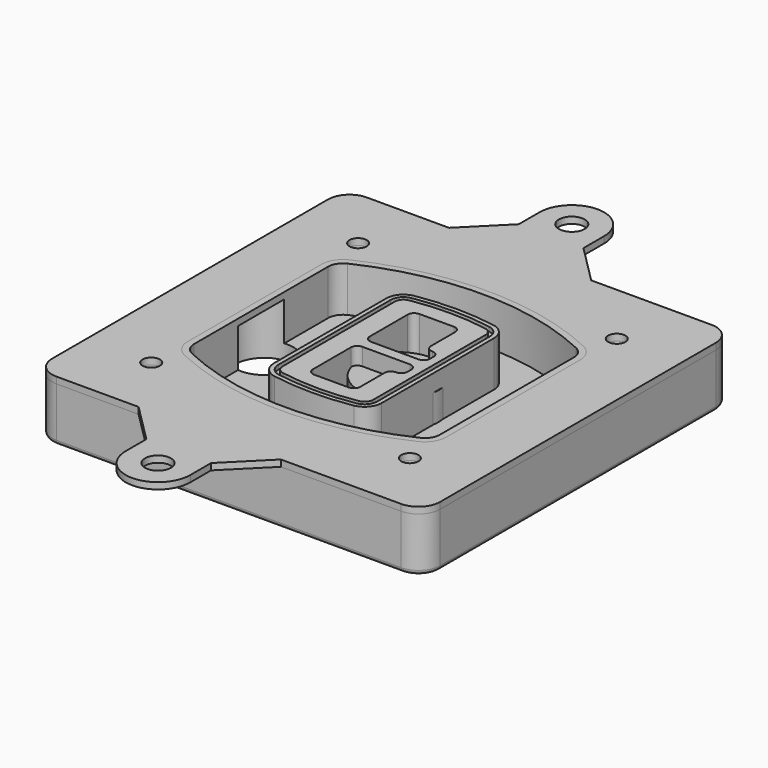
from build123d import *

# Parameters (mm, degrees)
F0_R      = 4
F1_DEPTH  = 25
F2_DEPTH  = 3
F3_DEPTH  = 18
F5_DEPTH  = 21
F6_DEPTH  = 2
F8_DEPTH  = 20
F9_DEPTH  = 16
F10_DEPTH = 25
F7_R      = 6
F7_R_2    = 4
F11_DEPTH = 6
F13_DEPTH = 9
F15_R     = 2
F16_R     = 4
F16_R_2   = 6
F17_DEPTH = 3


# Not quite as in the source:
# - a feature of the source that left no trace in its solid (it failed there, or was rolled back) is left out
# - a feature names something its author has since deleted; it is built from what else it names


with BuildPart() as f1:
    # F0 (on Top) → F1 (new body)
    with BuildSketch(Plane.XY):
        with BuildLine():
            ThreePointArc((-90, -80), (-87.0710678119, -87.0710678119), (-80, -90))
            Line((-80, -90), (80, -90))
            ThreePointArc((80, -90), (87.0710678119, -87.0710678119), (90, -80))
            Line((90, -80), (90, 80))
            ThreePointArc((90, 80), (87.0710678119, 87.0710678119), (80, 90))
            Line((80, 90), (-80, 90))
            ThreePointArc((-80, 90), (-87.0710678119, 87.0710678119), (-90, 80))
            Line((-90, 80), (-90, -80))
        make_face()
        with Locations((-60, -60)):
            Circle(F0_R, mode=Mode.SUBTRACT)
        with Locations((60, -60)):
            Circle(F0_R, mode=Mode.SUBTRACT)
        with BuildLine():
            ThreePointArc((-64, 38.8308515907), (-61.8195654598, 46.3340424013), (-55.9574468085, 51.5000594398))
            ThreePointArc((-55.9574468085, 51.5000594398), (0, 64), (55.9574468085, 51.5000594398))
            ThreePointArc((55.9574468085, 51.5000594398), (61.8195654598, 46.3340424013), (64, 38.8308515907))
            Line((64, 38.8308515907), (64, -38.8308515907))
            ThreePointArc((64, -38.8308515907), (61.8195654598, -46.3340424013), (55.9574468085, -51.5000594398))
            ThreePointArc((55.9574468085, -51.5000594398), (0, -64), (-55.9574468085, -51.5000594398))
            ThreePointArc((-55.9574468085, -51.5000594398), (-61.8195654598, -46.3340424013), (-64, -38.8308515907))
            Line((-64, -38.8308515907), (-64, 38.8308515907))
        make_face(mode=Mode.SUBTRACT)
        with Locations((-60, 60)):
            Circle(F0_R, mode=Mode.SUBTRACT)
        with Locations((60, 60)):
            Circle(F0_R, mode=Mode.SUBTRACT)
        with BuildLine():
            ThreePointArc((55.9574468085, 51.5000594398), (0, 64), (-55.9574468085, 51.5000594398))
            ThreePointArc((-55.9574468085, 51.5000594398), (-61.8195654598, 46.3340424013), (-64, 38.8308515907))
            Line((-64, 38.8308515907), (-64, -38.8308515907))
            ThreePointArc((-64, -38.8308515907), (-61.8195654598, -46.3340424013), (-55.9574468085, -51.5000594398))
            ThreePointArc((-55.9574468085, -51.5000594398), (0, -64), (55.9574468085, -51.5000594398))
            ThreePointArc((55.9574468085, -51.5000594398), (61.8195654598, -46.3340424013), (64, -38.8308515907))
            Line((64, -38.8308515907), (64, 38.8308515907))
            ThreePointArc((64, 38.8308515907), (61.8195654598, 46.3340424013), (55.9574468085, 51.5000594398))
        make_face()
        with BuildLine():
            Line((-60, -38.8308515907), (-60, 38.8308515907))
            ThreePointArc((-60, 38.8308515907), (-58.442546757, 44.1902735983), (-54.2553191489, 47.8802857686))
            ThreePointArc((-54.2553191489, 47.8802857686), (0, 60), (54.2553191489, 47.8802857686))
            ThreePointArc((54.2553191489, 47.8802857686), (58.442546757, 44.1902735983), (60, 38.8308515907))
            Line((60, 38.8308515907), (60, -38.8308515907))
            ThreePointArc((60, -38.8308515907), (58.442546757, -44.1902735983), (54.2553191489, -47.8802857686))
            ThreePointArc((54.2553191489, -47.8802857686), (0, -60), (-54.2553191489, -47.8802857686))
            ThreePointArc((-54.2553191489, -47.8802857686), (-58.442546757, -44.1902735983), (-60, -38.8308515907))
        make_face(mode=Mode.SUBTRACT)
        with BuildLine():
            ThreePointArc((-54.2553191489, 47.8802857686), (-58.442546757, 44.1902735983), (-60, 38.8308515907))
            Line((-60, 38.8308515907), (-60, -38.8308515907))
            ThreePointArc((-60, -38.8308515907), (-58.442546757, -44.1902735983), (-54.2553191489, -47.8802857686))
            ThreePointArc((-54.2553191489, -47.8802857686), (0, -60), (54.2553191489, -47.8802857686))
            ThreePointArc((54.2553191489, -47.8802857686), (58.442546757, -44.1902735983), (60, -38.8308515907))
            Line((60, -38.8308515907), (60, 38.8308515907))
            ThreePointArc((60, 38.8308515907), (58.442546757, 44.1902735983), (54.2553191489, 47.8802857686))
            ThreePointArc((54.2553191489, 47.8802857686), (0, 60), (-54.2553191489, 47.8802857686))
        make_face()
        with BuildLine():
            ThreePointArc((52.9787234043, 45.1654555152), (55.9097827299, 42.582446996), (57, 38.8308515907))
            Line((57, 38.8308515907), (57, -38.8308515907))
            ThreePointArc((57, -38.8308515907), (55.9097827299, -42.582446996), (52.9787234043, -45.1654555152))
            ThreePointArc((52.9787234043, -45.1654555152), (0, -57), (-52.9787234043, -45.1654555152))
            ThreePointArc((-52.9787234043, -45.1654555152), (-55.9097827299, -42.582446996), (-57, -38.8308515907))
            Line((-57, -38.8308515907), (-57, 38.8308515907))
            ThreePointArc((-57, 38.8308515907), (-55.9097827299, 42.582446996), (-52.9787234043, 45.1654555152))
            ThreePointArc((-52.9787234043, 45.1654555152), (0, 57), (52.9787234043, 45.1654555152))
        make_face(mode=Mode.SUBTRACT)
        with BuildLine():
            Line((57, -38.8308515907), (57, 38.8308515907))
            ThreePointArc((57, 38.8308515907), (55.9097827299, 42.582446996), (52.9787234043, 45.1654555152))
            ThreePointArc((52.9787234043, 45.1654555152), (0, 57), (-52.9787234043, 45.1654555152))
            ThreePointArc((-52.9787234043, 45.1654555152), (-55.9097827299, 42.582446996), (-57, 38.8308515907))
            Line((-57, 38.8308515907), (-57, -38.8308515907))
            ThreePointArc((-57, -38.8308515907), (-55.9097827299, -42.582446996), (-52.9787234043, -45.1654555152))
            ThreePointArc((-52.9787234043, -45.1654555152), (0, -57), (52.9787234043, -45.1654555152))
            ThreePointArc((52.9787234043, -45.1654555152), (55.9097827299, -42.582446996), (57, -38.8308515907))
        make_face()
    extrude(amount=-F1_DEPTH)

    # F0 (on Top) → F2 (join)
    with BuildSketch(Plane.XY):
        with BuildLine():
            ThreePointArc((-54.2553191489, 47.8802857686), (-58.442546757, 44.1902735983), (-60, 38.8308515907))
            Line((-60, 38.8308515907), (-60, -38.8308515907))
            ThreePointArc((-60, -38.8308515907), (-58.442546757, -44.1902735983), (-54.2553191489, -47.8802857686))
            ThreePointArc((-54.2553191489, -47.8802857686), (0, -60), (54.2553191489, -47.8802857686))
            ThreePointArc((54.2553191489, -47.8802857686), (58.442546757, -44.1902735983), (60, -38.8308515907))
            Line((60, -38.8308515907), (60, 38.8308515907))
            ThreePointArc((60, 38.8308515907), (58.442546757, 44.1902735983), (54.2553191489, 47.8802857686))
            ThreePointArc((54.2553191489, 47.8802857686), (0, 60), (-54.2553191489, 47.8802857686))
        make_face()
        with BuildLine():
            ThreePointArc((52.9787234043, 45.1654555152), (55.9097827299, 42.582446996), (57, 38.8308515907))
            Line((57, 38.8308515907), (57, -38.8308515907))
            ThreePointArc((57, -38.8308515907), (55.9097827299, -42.582446996), (52.9787234043, -45.1654555152))
            ThreePointArc((52.9787234043, -45.1654555152), (0, -57), (-52.9787234043, -45.1654555152))
            ThreePointArc((-52.9787234043, -45.1654555152), (-55.9097827299, -42.582446996), (-57, -38.8308515907))
            Line((-57, -38.8308515907), (-57, 38.8308515907))
            ThreePointArc((-57, 38.8308515907), (-55.9097827299, 42.582446996), (-52.9787234043, 45.1654555152))
            ThreePointArc((-52.9787234043, 45.1654555152), (0, 57), (52.9787234043, 45.1654555152))
        make_face(mode=Mode.SUBTRACT)
    extrude(amount=F2_DEPTH)

    # F0 (on Top) → F3 (cut)
    with BuildSketch(Plane.XY):
        with BuildLine():
            Line((57, -38.8308515907), (57, 38.8308515907))
            ThreePointArc((57, 38.8308515907), (55.9097827299, 42.582446996), (52.9787234043, 45.1654555152))
            ThreePointArc((52.9787234043, 45.1654555152), (0, 57), (-52.9787234043, 45.1654555152))
            ThreePointArc((-52.9787234043, 45.1654555152), (-55.9097827299, 42.582446996), (-57, 38.8308515907))
            Line((-57, 38.8308515907), (-57, -38.8308515907))
            ThreePointArc((-57, -38.8308515907), (-55.9097827299, -42.582446996), (-52.9787234043, -45.1654555152))
            ThreePointArc((-52.9787234043, -45.1654555152), (0, -57), (52.9787234043, -45.1654555152))
            ThreePointArc((52.9787234043, -45.1654555152), (55.9097827299, -42.582446996), (57, -38.8308515907))
        make_face()
    extrude(amount=-F3_DEPTH, mode=Mode.SUBTRACT)

    # F4 (on face) → F5 (join, through all)
    with BuildSketch(Plane.XY.offset(3)):
        with BuildLine():
            ThreePointArc((-25, -32.5662280692), (-23.1122504785, -37.7276614059), (-18.3399014778, -40.4532214146))
            ThreePointArc((-18.3399014778, -40.4532214146), (0, -42), (18.3399014778, -40.4532214146))
            ThreePointArc((18.3399014778, -40.4532214146), (23.1122504785, -37.7276614059), (25, -32.5662280692))
            Line((25, -32.5662280692), (25, 32.5662280692))
            ThreePointArc((25, 32.5662280692), (23.1122504785, 37.7276614059), (18.3399014778, 40.4532214146))
            ThreePointArc((18.3399014778, 40.4532214146), (0, 42), (-18.3399014778, 40.4532214146))
            ThreePointArc((-18.3399014778, 40.4532214146), (-23.1122504785, 37.7276614059), (-25, 32.5662280692))
            Line((-25, 32.5662280692), (-25, -32.5662280692))
        make_face()
        with BuildLine():
            ThreePointArc((18.0049261084, 38.4814730782), (21.5841878588, 36.4373030717), (23, 32.5662280692))
            Line((23, 32.5662280692), (23, -32.5662280692))
            ThreePointArc((23, -32.5662280692), (21.5841878588, -36.4373030717), (18.0049261084, -38.4814730782))
            ThreePointArc((18.0049261084, -38.4814730782), (0, -40), (-18.0049261084, -38.4814730782))
            ThreePointArc((-18.0049261084, -38.4814730782), (-21.5841878588, -36.4373030717), (-23, -32.5662280692))
            Line((-23, -32.5662280692), (-23, 32.5662280692))
            ThreePointArc((-23, 32.5662280692), (-21.5841878588, 36.4373030717), (-18.0049261084, 38.4814730782))
            ThreePointArc((-18.0049261084, 38.4814730782), (0, 40), (18.0049261084, 38.4814730782))
        make_face(mode=Mode.SUBTRACT)
        with BuildLine():
            Line((23, -32.5662280692), (23, 32.5662280692))
            ThreePointArc((23, 32.5662280692), (21.5841878588, 36.4373030717), (18.0049261084, 38.4814730782))
            ThreePointArc((18.0049261084, 38.4814730782), (0, 40), (-18.0049261084, 38.4814730782))
            ThreePointArc((-18.0049261084, 38.4814730782), (-21.5841878588, 36.4373030717), (-23, 32.5662280692))
            Line((-23, 32.5662280692), (-23, -32.5662280692))
            ThreePointArc((-23, -32.5662280692), (-21.5841878588, -36.4373030717), (-18.0049261084, -38.4814730782))
            ThreePointArc((-18.0049261084, -38.4814730782), (0, -40), (18.0049261084, -38.4814730782))
            ThreePointArc((18.0049261084, -38.4814730782), (21.5841878588, -36.4373030717), (23, -32.5662280692))
        make_face()
        with BuildLine():
            ThreePointArc((17.6699507389, 36.5097247419), (20.0561252392, 35.1469447375), (21, 32.5662280692))
            Line((21, 32.5662280692), (21, -32.5662280692))
            ThreePointArc((21, -32.5662280692), (20.0561252392, -35.1469447375), (17.6699507389, -36.5097247419))
            ThreePointArc((17.6699507389, -36.5097247419), (0, -38), (-17.6699507389, -36.5097247419))
            ThreePointArc((-17.6699507389, -36.5097247419), (-20.0561252392, -35.1469447375), (-21, -32.5662280692))
            Line((-21, -32.5662280692), (-21, 32.5662280692))
            ThreePointArc((-21, 32.5662280692), (-20.0561252392, 35.1469447375), (-17.6699507389, 36.5097247419))
            ThreePointArc((-17.6699507389, 36.5097247419), (0, 38), (17.6699507389, 36.5097247419))
        make_face(mode=Mode.SUBTRACT)
        with BuildLine():
            Line((21, -32.5662280692), (21, 32.5662280692))
            ThreePointArc((21, 32.5662280692), (20.0561252392, 35.1469447375), (17.6699507389, 36.5097247419))
            ThreePointArc((17.6699507389, 36.5097247419), (0, 38), (-17.6699507389, 36.5097247419))
            ThreePointArc((-17.6699507389, 36.5097247419), (-20.0561252392, 35.1469447375), (-21, 32.5662280692))
            Line((-21, 32.5662280692), (-21, -32.5662280692))
            ThreePointArc((-21, -32.5662280692), (-20.0561252392, -35.1469447375), (-17.6699507389, -36.5097247419))
            ThreePointArc((-17.6699507389, -36.5097247419), (0, -38), (17.6699507389, -36.5097247419))
            ThreePointArc((17.6699507389, -36.5097247419), (20.0561252392, -35.1469447375), (21, -32.5662280692))
        make_face()
        with BuildLine():
            Line((-8, -2.5), (14, -2.5))
            ThreePointArc((14, -2.5), (16.1213203436, -3.3786796564), (17, -5.5))
            Line((17, -5.5), (17, -7.5))
            ThreePointArc((17, -7.5), (16.1213203436, -9.6213203436), (14, -10.5))
            ThreePointArc((14, -10.5), (11.8786796564, -11.3786796564), (11, -13.5))
            Line((11, -13.5), (11, -27.5))
            ThreePointArc((11, -27.5), (10.1213203436, -29.6213203436), (8, -30.5))
            Line((8, -30.5), (-8, -30.5))
            ThreePointArc((-8, -30.5), (-10.1213203436, -29.6213203436), (-11, -27.5))
            Line((-11, -27.5), (-11, -5.5))
            ThreePointArc((-11, -5.5), (-10.1213203436, -3.3786796564), (-8, -2.5))
        make_face(mode=Mode.SUBTRACT)
        with BuildLine():
            ThreePointArc((-8, 2.5), (-10.1213203436, 3.3786796564), (-11, 5.5))
            Line((-11, 5.5), (-11, 27.5))
            ThreePointArc((-11, 27.5), (-10.1213203436, 29.6213203436), (-8, 30.5))
            Line((-8, 30.5), (8, 30.5))
            ThreePointArc((8, 30.5), (10.1213203436, 29.6213203436), (11, 27.5))
            Line((11, 27.5), (11, 13.5))
            ThreePointArc((11, 13.5), (11.8786796564, 11.3786796564), (14, 10.5))
            ThreePointArc((14, 10.5), (16.1213203436, 9.6213203436), (17, 7.5))
            Line((17, 7.5), (17, 5.5))
            ThreePointArc((17, 5.5), (16.1213203436, 3.3786796564), (14, 2.5))
            Line((14, 2.5), (-8, 2.5))
        make_face(mode=Mode.SUBTRACT)
    extrude(amount=-F5_DEPTH)

    # F4 (on face) → F6 (cut)
    with BuildSketch(Plane.XY.offset(3)):
        with BuildLine():
            Line((23, -32.5662280692), (23, 32.5662280692))
            ThreePointArc((23, 32.5662280692), (21.5841878588, 36.4373030717), (18.0049261084, 38.4814730782))
            ThreePointArc((18.0049261084, 38.4814730782), (0, 40), (-18.0049261084, 38.4814730782))
            ThreePointArc((-18.0049261084, 38.4814730782), (-21.5841878588, 36.4373030717), (-23, 32.5662280692))
            Line((-23, 32.5662280692), (-23, -32.5662280692))
            ThreePointArc((-23, -32.5662280692), (-21.5841878588, -36.4373030717), (-18.0049261084, -38.4814730782))
            ThreePointArc((-18.0049261084, -38.4814730782), (0, -40), (18.0049261084, -38.4814730782))
            ThreePointArc((18.0049261084, -38.4814730782), (21.5841878588, -36.4373030717), (23, -32.5662280692))
        make_face()
        with BuildLine():
            ThreePointArc((17.6699507389, 36.5097247419), (20.0561252392, 35.1469447375), (21, 32.5662280692))
            Line((21, 32.5662280692), (21, -32.5662280692))
            ThreePointArc((21, -32.5662280692), (20.0561252392, -35.1469447375), (17.6699507389, -36.5097247419))
            ThreePointArc((17.6699507389, -36.5097247419), (0, -38), (-17.6699507389, -36.5097247419))
            ThreePointArc((-17.6699507389, -36.5097247419), (-20.0561252392, -35.1469447375), (-21, -32.5662280692))
            Line((-21, -32.5662280692), (-21, 32.5662280692))
            ThreePointArc((-21, 32.5662280692), (-20.0561252392, 35.1469447375), (-17.6699507389, 36.5097247419))
            ThreePointArc((-17.6699507389, 36.5097247419), (0, 38), (17.6699507389, 36.5097247419))
        make_face(mode=Mode.SUBTRACT)
    extrude(amount=-F6_DEPTH, mode=Mode.SUBTRACT)

    # F7 (on face) → F8 (join)
    with BuildSketch(Plane(origin=(0, 0, -25), x_dir=(1, 0, 0), z_dir=(0, 0, -1))):
        with BuildLine():
            ThreePointArc((-6.71157564, 0), (6.7567035675, 13.4682792075), (20.224982775, 0))
            Line((20.224982775, 0), (25.224982775, 0))
            ThreePointArc((25.224982775, 0), (6.7567035675, 18.4682792075), (-11.71157564, 0))
            Line((-11.71157564, 0), (-6.71157564, 0))
        make_face()
        with BuildLine():
            Line((-6.71157564, 0), (20.224982775, 0))
            ThreePointArc((20.224982775, 0), (6.7567035675, 13.4682792075), (-6.71157564, 0))
        make_face()
        with BuildLine():
            ThreePointArc((-6.71157564, 0), (6.7567035675, -13.4682792075), (20.224982775, 0))
            Line((20.224982775, 0), (-6.71157564, 0))
        make_face()
        with BuildLine():
            Line((25.224982775, 0), (20.224982775, 0))
            ThreePointArc((20.224982775, 0), (6.7567035675, -13.4682792075), (-6.71157564, 0))
            Line((-6.71157564, 0), (-11.71157564, 0))
            ThreePointArc((-11.71157564, 0), (6.7567035675, -18.4682792075), (25.224982775, 0))
        make_face()
    extrude(amount=-F8_DEPTH)

    # F7 (on face) → F9 (cut)
    with BuildSketch(Plane(origin=(0, 0, -25), x_dir=(1, 0, 0), z_dir=(0, 0, -1))):
        with BuildLine():
            Line((-6.71157564, 0), (20.224982775, 0))
            ThreePointArc((20.224982775, 0), (6.7567035675, 13.4682792075), (-6.71157564, 0))
        make_face()
        with BuildLine():
            ThreePointArc((-6.71157564, 0), (6.7567035675, -13.4682792075), (20.224982775, 0))
            Line((20.224982775, 0), (-6.71157564, 0))
        make_face()
    extrude(amount=-F9_DEPTH, mode=Mode.SUBTRACT)

    # F7 (on face) → F10 (cut)
    with BuildSketch(Plane(origin=(0, 0, -25), x_dir=(1, 0, 0), z_dir=(0, 0, -1))):
        with BuildLine():
            Line((-69.0318229325, 0), (-42.0952645175, 0))
            ThreePointArc((-42.0952645175, 0), (-55.563543725, 13.4682792075), (-69.0318229325, 0))
        make_face()
        with BuildLine():
            ThreePointArc((-69.0318229325, 0), (-55.563543725, -13.4682792075), (-42.0952645175, 0))
            Line((-42.0952645175, 0), (-69.0318229325, 0))
        make_face()
    extrude(amount=-F10_DEPTH, mode=Mode.SUBTRACT)

    # F7 (on face) → F11 (cut)
    with BuildSketch(Plane(origin=(0, 0, -25), x_dir=(1, 0, 0), z_dir=(0, 0, -1))):
        with Locations((60, -60)):
            Circle(F7_R)
        with Locations((60, -60)):
            Circle(F7_R_2, mode=Mode.SUBTRACT)
        with Locations((-60, -60)):
            Circle(F7_R)
        with Locations((-60, -60)):
            Circle(F7_R_2, mode=Mode.SUBTRACT)
        with Locations((-60, 60)):
            Circle(F7_R)
        with Locations((-60, 60)):
            Circle(F7_R_2, mode=Mode.SUBTRACT)
        with Locations((60, 60)):
            Circle(F7_R)
        with Locations((60, 60)):
            Circle(F7_R_2, mode=Mode.SUBTRACT)
    extrude(amount=-F11_DEPTH, mode=Mode.SUBTRACT)

    # F12 (on face) → F13 (cut, through all)
    with BuildSketch(Plane(origin=(0, 0, -9), x_dir=(1, 0, 0), z_dir=(0, 0, -1))):
        with BuildLine():
            ThreePointArc((20.224982775, 0), (20.1663399806, 1.2554664788), (19.9909222755, 2.5))
            Line((19.9909222755, 2.5), (14, 2.5))
            ThreePointArc((14, 2.5), (16.1213203436, 3.3786796564), (17, 5.5))
            Line((17, 5.5), (17, 7.5))
            ThreePointArc((17, 7.5), (16.1213203436, 9.6213203436), (14, 10.5))
            ThreePointArc((14, 10.5), (12.1627255951, 11.1284134507), (11.0951631559, 12.750384826))
            ThreePointArc((11.0951631559, 12.750384826), (11.0476113807, 12.7664660322), (11, 12.7823698976))
            Line((11, 12.7823698976), (11, -12.7823698976))
            ThreePointArc((11, -12.7823698976), (11.0476113807, -12.7664660322), (11.0951631559, -12.750384826))
            ThreePointArc((11.0951631559, -12.750384826), (12.1627255951, -11.1284134507), (14, -10.5))
            ThreePointArc((14, -10.5), (16.1213203436, -9.6213203436), (17, -7.5))
            Line((17, -7.5), (17, -5.5))
            ThreePointArc((17, -5.5), (16.1213203436, -3.3786796564), (14, -2.5))
            Line((14, -2.5), (19.9909222755, -2.5))
            ThreePointArc((19.9909222755, -2.5), (20.1663399806, -1.2554664788), (20.224982775, 0))
        make_face()
    extrude(amount=F13_DEPTH, mode=Mode.SUBTRACT)

    # F15
    f15_edges = [f1.edges().sort_by_distance(p)[0] for p in [
        (0, -90, -25),
        (-87.071068, -87.071068, -25),
        (-90, 0, -25),
        (-87.071068, 87.071068, -25),
        (87.071068, -87.071068, -25),
        (0, 90, -25),
        (90, 0, -25),
        (87.071068, 87.071068, -25),
    ]]
    fillet(f15_edges, radius=F15_R)


with BuildPart() as f17:
    # F16 (on Top) → F17 (new body, through all)
    with BuildSketch(Plane.XY):
        with BuildLine():
            Line((-90, 80), (-90, -80))
            ThreePointArc((-90, -80), (-87.0710678119, -87.0710678119), (-80, -90))
            Line((-80, -90), (-41.8600961566, -90))
            Line((-41.8600961566, -90), (24.1399038434, -90))
            Line((24.1399038434, -90), (80, -90))
            ThreePointArc((80, -90), (87.0710678119, -87.0710678119), (90, -80))
            Line((90, -80), (90, 80))
            ThreePointArc((90, 80), (87.0710678119, 87.0710678119), (80, 90))
            Line((80, 90), (24.1399038434, 90))
            Line((24.1399038434, 90), (-41.8600961566, 90))
            Line((-41.8600961566, 90), (-80, 90))
            ThreePointArc((-80, 90), (-87.0710678119, 87.0710678119), (-90, 80))
        make_face()
        with Locations((-60, -60)):
            Circle(F16_R, mode=Mode.SUBTRACT)
        with Locations((60, -60)):
            Circle(F16_R, mode=Mode.SUBTRACT)
        with Locations((-60, 60)):
            Circle(F16_R, mode=Mode.SUBTRACT)
        with BuildLine():
            ThreePointArc((-54.2553191489, 47.8802857686), (0, 60), (54.2553191489, 47.8802857686))
            ThreePointArc((54.2553191489, 47.8802857686), (58.442546757, 44.1902735983), (60, 38.8308515907))
            Line((60, 38.8308515907), (60, -38.8308515907))
            ThreePointArc((60, -38.8308515907), (58.442546757, -44.1902735983), (54.2553191489, -47.8802857686))
            ThreePointArc((54.2553191489, -47.8802857686), (0, -60), (-54.2553191489, -47.8802857686))
            ThreePointArc((-54.2553191489, -47.8802857686), (-58.442546757, -44.1902735983), (-60, -38.8308515907))
            Line((-60, -38.8308515907), (-60, 38.8308515907))
            ThreePointArc((-60, 38.8308515907), (-58.442546757, 44.1902735983), (-54.2553191489, 47.8802857686))
        make_face(mode=Mode.SUBTRACT)
        with Locations((60, 60)):
            Circle(F16_R, mode=Mode.SUBTRACT)
        with BuildLine():
            Line((24.1399038434, -90), (-41.8600961566, -90))
            Line((-41.8600961566, -90), (-23.8600961566, -108))
            Line((-23.8600961566, -108), (-23.8600961566, -120))
            ThreePointArc((-23.8600961566, -120), (-8.8600961566, -135), (6.1399038434, -120))
            Line((6.1399038434, -120), (6.1399038434, -108))
            Line((6.1399038434, -108), (24.1399038434, -90))
        make_face()
        with Locations((-8.8600961566, -120)):
            Circle(F16_R_2, mode=Mode.SUBTRACT)
        with BuildLine():
            Line((-23.8600961566, 108), (-41.8600961566, 90))
            Line((-41.8600961566, 90), (24.1399038434, 90))
            Line((24.1399038434, 90), (6.1399038434, 108))
            Line((6.1399038434, 108), (6.1399038434, 120))
            ThreePointArc((6.1399038434, 120), (-8.8600961566, 135), (-23.8600961566, 120))
            Line((-23.8600961566, 120), (-23.8600961566, 108))
        make_face()
        with Locations((-8.8600961566, 120)):
            Circle(F16_R_2, mode=Mode.SUBTRACT)
    extrude(amount=F17_DEPTH)


solid = Compound([f1.part, f17.part])
